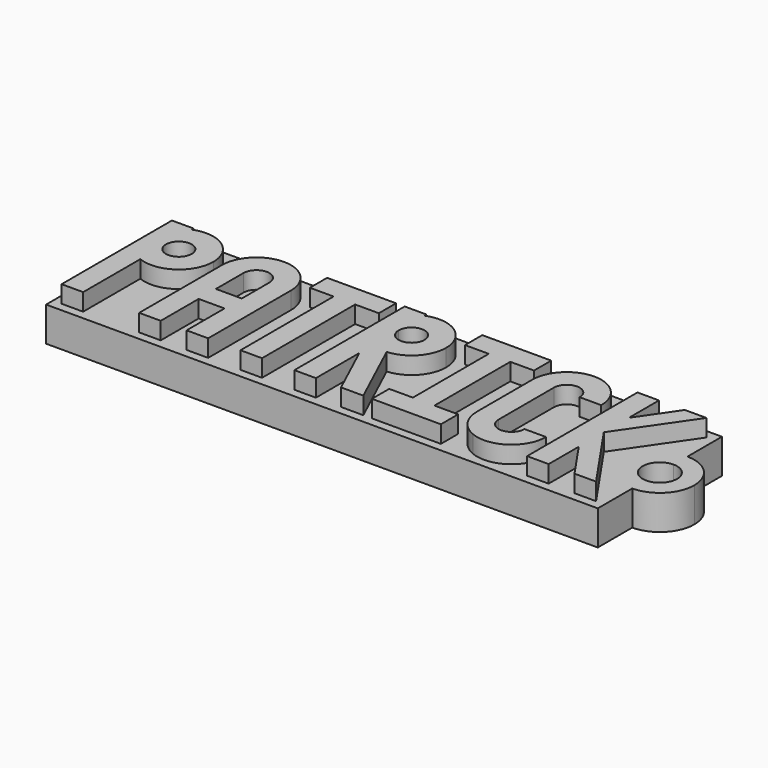
from build123d import *

# Parameters (mm, degrees)
F1_DEPTH = 4
F2_W     = 2.5
F2_H     = 2.5
F2_H_2   = 5.5
F2_W_2   = 2.75
F2_H_3   = 13.5
F2_H_4   = 11
F3_DEPTH = 2


with BuildPart() as f1:
    # F0 (on Top) → F1 (new body)
    with BuildSketch(Plane.XY):
        with BuildLine():
            Line((-64, 0), (0, 0))
            Line((0, 0), (0, 5))
            ThreePointArc((0, 5), (-4, 9), (0, 13))
            Line((0, 13), (0, 18))
            Line((0, 18), (-64, 18))
            Line((-64, 18), (-64, 0))
        make_face()
        with BuildLine():
            ThreePointArc((0, 13), (-4, 9), (0, 5))
            Line((0, 5), (0, 7))
            ThreePointArc((0, 7), (-2, 9), (0, 11))
            Line((0, 11), (0, 13))
        make_face()
        with BuildLine():
            Line((0, 7), (0, 5))
            ThreePointArc((0, 5), (2.8284271247, 6.1715728753), (4, 9))
            ThreePointArc((4, 9), (2.8284271247, 11.8284271247), (0, 13))
            Line((0, 13), (0, 11))
            ThreePointArc((0, 11), (1.4142135624, 10.4142135624), (2, 9))
            ThreePointArc((2, 9), (1.4142135624, 7.5857864376), (0, 7))
        make_face()
    extrude(amount=F1_DEPTH)

    # F2 (on face) → F3 (join)
    with BuildSketch(Plane.XY.offset(4)):
        with BuildLine():
            Line((-60.5, 17), (-63, 17))
            Line((-63, 17), (-63, 13))
            ThreePointArc((-63, 13), (-62.3166247904, 15.2360679775), (-60.5, 16.7080992435))
            Line((-60.5, 16.7080992435), (-60.5, 17))
        make_face()
        with BuildLine():
            ThreePointArc((-60.5, 9.2919007565), (-62.3166247904, 10.7639320225), (-63, 13))
            Line((-63, 13), (-63, 1))
            Line((-63, 1), (-60.5, 1))
            Line((-60.5, 1), (-60.5, 9.2919007565))
        make_face()
        with BuildLine():
            ThreePointArc((-60.5, 16.7080992435), (-62.3166247904, 15.2360679775), (-63, 13))
            ThreePointArc((-63, 13), (-62.3166247904, 10.7639320225), (-60.5, 9.2919007565))
            Line((-60.5, 9.2919007565), (-60.5, 13))
            Line((-60.5, 13), (-60.5, 16.7080992435))
        make_face()
        with BuildLine():
            ThreePointArc((-55, 13), (-56.7639320225, 16.3166247904), (-60.5, 16.7080992435))
            Line((-60.5, 16.7080992435), (-60.5, 13))
            Line((-60.5, 13), (-60.5, 9.2919007565))
            ThreePointArc((-60.5, 9.2919007565), (-56.7639320225, 9.6833752096), (-55, 13))
        make_face()
        with BuildLine():
            ThreePointArc((-57.5, 13), (-59, 11.5), (-60.5, 13))
            ThreePointArc((-60.5, 13), (-59, 14.5), (-57.5, 13))
        make_face(mode=Mode.SUBTRACT)
        with Locations((-52.75, 7.75)):
            Rectangle(F2_W, F2_H)
        with BuildLine():
            Line((-54, 13), (-54, 9))
            Line((-54, 9), (-51.5, 9))
            Line((-51.5, 9), (-51.5, 9.2919007565))
            ThreePointArc((-51.5, 9.2919007565), (-53.3166247904, 10.7639320225), (-54, 13))
        make_face()
        with Locations((-52.75, 3.75)):
            Rectangle(F2_W, F2_H_2)
        with BuildLine():
            ThreePointArc((-51.5, 16.7080992435), (-53.3166247904, 15.2360679775), (-54, 13))
            ThreePointArc((-54, 13), (-53.3166247904, 10.7639320225), (-51.5, 9.2919007565))
            Line((-51.5, 9.2919007565), (-51.5, 13))
            Line((-51.5, 13), (-51.5, 16.7080992435))
        make_face()
        Polygon((-50, 9), (-51.5, 9), (-51.5, 6.5), (-48.5, 6.5), (-48.5, 9), align=None)
        with BuildLine():
            ThreePointArc((-48.5, 16.7080992435), (-50, 17), (-51.5, 16.7080992435))
            Line((-51.5, 16.7080992435), (-51.5, 13))
            ThreePointArc((-51.5, 13), (-50, 14.5), (-48.5, 13))
            Line((-48.5, 13), (-48.5, 16.7080992435))
        make_face()
        with Locations((-47.25, 3.75)):
            Rectangle(F2_W, F2_H_2)
        with Locations((-47.25, 7.75)):
            Rectangle(F2_W, F2_H)
        with BuildLine():
            ThreePointArc((-46, 13), (-46.6833752096, 15.2360679775), (-48.5, 16.7080992435))
            Line((-48.5, 16.7080992435), (-48.5, 13))
            Line((-48.5, 13), (-48.5, 9.2919007565))
            ThreePointArc((-48.5, 9.2919007565), (-46.6833752096, 10.7639320225), (-46, 13))
        make_face()
        with BuildLine():
            Line((-48.5, 9.2919007565), (-48.5, 9))
            Line((-48.5, 9), (-46, 9))
            Line((-46, 9), (-46, 13))
            ThreePointArc((-46, 13), (-46.6833752096, 10.7639320225), (-48.5, 9.2919007565))
        make_face()
        with Locations((-43.625, 15.75)):
            Rectangle(F2_W_2, F2_H)
        with Locations((-41, 15.75)):
            Rectangle(F2_W, F2_H)
        with Locations((-38.375, 15.75)):
            Rectangle(F2_W_2, F2_H)
        with Locations((-41, 7.75)):
            Rectangle(F2_W, F2_H_3)
        with BuildLine():
            Line((-33.5, 17), (-36, 17))
            Line((-36, 17), (-36, 13))
            ThreePointArc((-36, 13), (-35.3166247904, 15.2360679775), (-33.5, 16.7080992435))
            Line((-33.5, 16.7080992435), (-33.5, 17))
        make_face()
        with BuildLine():
            ThreePointArc((-34.8284271247, 10.1715728753), (-35.69551813, 11.4692662705), (-36, 13))
            Line((-36, 13), (-36, 1))
            Line((-36, 1), (-33.5, 1))
            Line((-33.5, 1), (-33.5, 7.299987892))
            Line((-33.5, 7.299987892), (-34.8284271247, 10.1715728753))
        make_face()
        with BuildLine():
            ThreePointArc((-33.5, 16.7080992435), (-35.3166247904, 15.2360679775), (-36, 13))
            ThreePointArc((-36, 13), (-35.69551813, 11.4692662705), (-34.8284271247, 10.1715728753))
            ThreePointArc((-34.8284271247, 10.1715728753), (-34.2084555922, 9.6649252036), (-33.5, 9.2919007565))
            Line((-33.5, 9.2919007565), (-33.5, 13))
            Line((-33.5, 13), (-33.5, 16.7080992435))
        make_face()
        with BuildLine():
            ThreePointArc((-28, 13), (-29.7639320225, 16.3166247904), (-33.5, 16.7080992435))
            Line((-33.5, 16.7080992435), (-33.5, 13))
            ThreePointArc((-33.5, 13), (-32, 14.5), (-30.5, 13))
            ThreePointArc((-30.5, 13), (-31.4259748515, 11.6141807012), (-33.0606601718, 11.9393398282))
            Line((-33.0606601718, 11.9393398282), (-31.7058974503, 9.0108266909))
            ThreePointArc((-31.7058974503, 9.0108266909), (-29.0694360441, 10.2775388156), (-28, 13))
        make_face()
        with BuildLine():
            ThreePointArc((-33.5, 9.2919007565), (-34.2084555922, 9.6649252036), (-34.8284271247, 10.1715728753))
            Line((-34.8284271247, 10.1715728753), (-33.5, 7.299987892))
            Line((-33.5, 7.299987892), (-33.5, 9.2919007565))
        make_face()
        with BuildLine():
            ThreePointArc((-33.0606601718, 11.9393398282), (-33.3858192988, 12.4259748515), (-33.5, 13))
            Line((-33.5, 13), (-33.5, 9.2919007565))
            ThreePointArc((-33.5, 9.2919007565), (-32.6191105093, 9.048202665), (-31.7058974503, 9.0108266909))
            Line((-31.7058974503, 9.0108266909), (-33.0606601718, 11.9393398282))
        make_face()
        with BuildLine():
            ThreePointArc((-31.7058974503, 9.0108266909), (-32.6191105093, 9.048202665), (-33.5, 9.2919007565))
            Line((-33.5, 9.2919007565), (-33.5, 7.299987892))
            Line((-33.5, 7.299987892), (-30.5855555903, 1))
            Line((-30.5855555903, 1), (-28, 1))
            Line((-28, 1), (-31.7058974503, 9.0108266909))
        make_face()
        with Locations((-25.625, 15.75)):
            Rectangle(F2_W_2, F2_H)
        with Locations((-23, 15.75)):
            Rectangle(F2_W, F2_H)
        with Locations((-20.375, 15.75)):
            Rectangle(F2_W_2, F2_H)
        with Locations((-23, 9)):
            Rectangle(F2_W, F2_H_4)
        with Locations((-25.625, 2.25)):
            Rectangle(F2_W_2, F2_H)
        with Locations((-23, 2.25)):
            Rectangle(F2_W, F2_H)
        with Locations((-20.375, 2.25)):
            Rectangle(F2_W_2, F2_H)
        with BuildLine():
            ThreePointArc((-15.5, 9.2919007565), (-17.3166247904, 10.7639320225), (-18, 13))
            Line((-18, 13), (-18, 5))
            ThreePointArc((-18, 5), (-17.3166247904, 7.2360679775), (-15.5, 8.7080992435))
            Line((-15.5, 8.7080992435), (-15.5, 9.2919007565))
        make_face()
        with BuildLine():
            ThreePointArc((-15.5, 16.7080992435), (-17.3166247904, 15.2360679775), (-18, 13))
            ThreePointArc((-18, 13), (-17.3166247904, 10.7639320225), (-15.5, 9.2919007565))
            Line((-15.5, 9.2919007565), (-15.5, 13))
            Line((-15.5, 13), (-15.5, 16.7080992435))
        make_face()
        with BuildLine():
            ThreePointArc((-15.5, 8.7080992435), (-17.3166247904, 7.2360679775), (-18, 5))
            ThreePointArc((-18, 5), (-17.3166247904, 2.7639320225), (-15.5, 1.2919007565))
            Line((-15.5, 1.2919007565), (-15.5, 5))
            Line((-15.5, 5), (-15.5, 8.7080992435))
        make_face()
        with BuildLine():
            ThreePointArc((-10, 13), (-11.7639320225, 16.3166247904), (-15.5, 16.7080992435))
            Line((-15.5, 16.7080992435), (-15.5, 13))
            ThreePointArc((-15.5, 13), (-14, 14.5), (-12.5, 13))
            Line((-12.5, 13), (-10, 13))
        make_face()
        with BuildLine():
            Line((-15.5, 5), (-15.5, 1.2919007565))
            ThreePointArc((-15.5, 1.2919007565), (-11.7639320225, 1.6833752096), (-10, 5))
            Line((-10, 5), (-12.5, 5))
            ThreePointArc((-12.5, 5), (-14, 3.5), (-15.5, 5))
        make_face()
        Polygon((-6.5, 17), (-9, 17), (-9, 9), (-6.5, 12.6363636364), align=None)
        Polygon((-6.5, 5.3636363636), (-9, 9), (-9, 1), (-6.5, 1), align=None)
        Polygon((-6.5, 12.6363636364), (-9, 9), (-6.5, 5.3636363636), (-6.5, 9), align=None)
        Polygon((-3.5, 17), (-6.5, 12.6363636364), (-6.5, 9), (-1, 17), align=None)
        Polygon((-6.5, 9), (-6.5, 5.3636363636), (-3.5, 1), (-1, 1), align=None)
    extrude(amount=F3_DEPTH)


solid = f1.part
